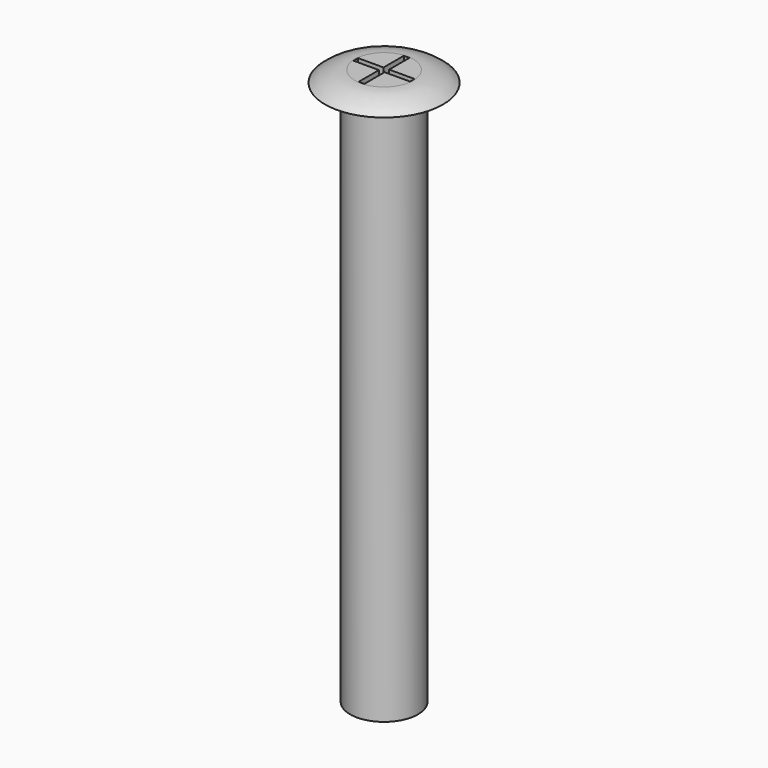
from build123d import *

# Parameters (mm, degrees)
F0_R     = 1.5
F1_DEPTH = 24.6
F2_R     = 2.61
F2_R_2   = 1.5
F3_DEPTH = 0.5
F5_DEPTH = 0.5


# Not quite as in the source:
# - a fillet or chamfer that OpenCascade refuses, or shapes differently, is made with other operations: its cross-section is extruded or revolved along the edge and cut away or added


with BuildPart() as f1:
    # F0 (on Top) → F1 (new body)
    with BuildSketch(Plane.XY):
        Circle(F0_R)
    extrude(amount=F1_DEPTH)

    # F2 (on face) → F3 (join)
    with BuildSketch(Plane.XY.offset(24.6)):
        Circle(F2_R)
        Circle(F2_R_2, mode=Mode.SUBTRACT)
    extrude(amount=-F3_DEPTH)

    # F4: fillet of radius 2 on 1 edges, made by hand

    # F4_s1 → F4_t2 (revolve, cut)
    with BuildSketch(Plane.XZ):
        with BuildLine():
            ThreePointArc((2.61, 24.1), (1.9942311257, 24.4708286934), (1.2871243445, 24.6))
            Line((1.2871243445, 24.6), (2.61, 24.6))
            Line((2.61, 24.6), (2.61, 24.1))
        make_face()
    revolve(axis=Axis((0, 0, 24.6), (0, 0, 1)), mode=Mode.SUBTRACT)

    # F2 (on face) → F5 (cut)
    with BuildSketch(Plane.XY.offset(24.6)):
        Polygon((-1.2485300168, 0.125), (-1.2485300168, -0.125), (-0.125, -0.125), (-0.125, -1.2485300168), (0.125, -1.2485300168), (0.125, -0.125), (1.2485300168, -0.125), (1.2485300168, 0.125), (0.125, 0.125), (0.125, 1.2485300168), (-0.125, 1.2485300168), (-0.125, 0.125), align=None)
    extrude(amount=-F5_DEPTH, mode=Mode.SUBTRACT)


solid = f1.part
